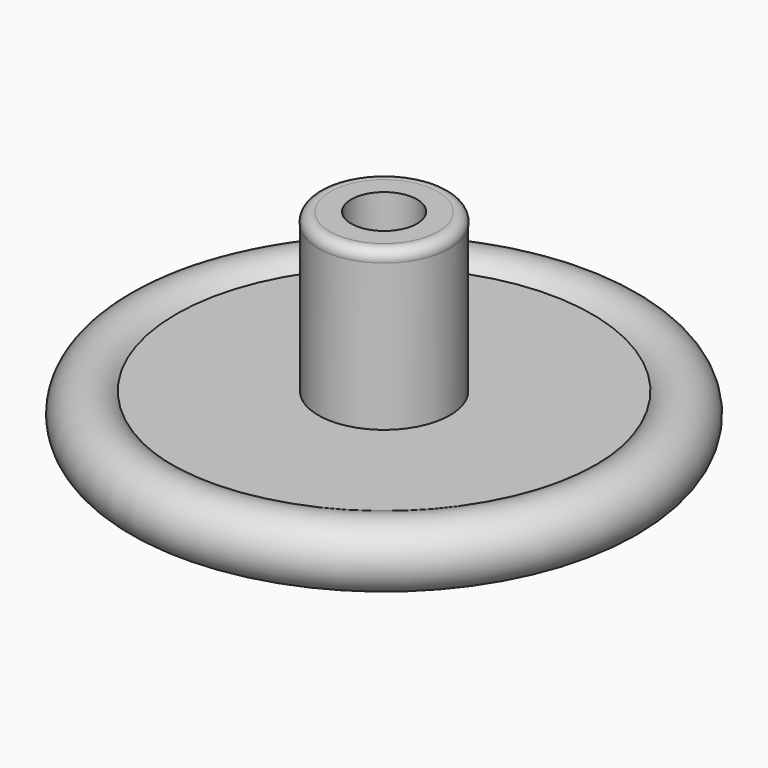
from build123d import *

# Parameters (mm, degrees)
F2_R     = 3.96875
F3_DEPTH = 9.525
F4_R     = 1.5875
F5_DEPTH = 20.6375


# Not quite as in the source:
# - a length typed as a fraction of an inch, garbled in the dataset ("3 / 203.2 mm" for 3/8 in), is restored


with BuildPart() as f1:
    # F0 (on Front) → F1 (revolve)
    with BuildSketch(Plane.XZ):
        with BuildLine():
            Line((0, 30.1625), (0, 0))
            Line((0, 0), (5.2339527756, 0))
            ThreePointArc((5.2339527756, 0), (6.9300739719, 1.2963017107), (7.94385, 3.17499365))
            Line((7.94385, 3.17499365), (7.9375, 6.3499873))
            Line((7.9375, 6.3499873), (25.0110084837, 6.3499873))
            ThreePointArc((25.0110084837, 6.3499873), (31.8322699863, 8.6224170081), (25.0874177301, 11.1125))
            Line((25.0874177301, 11.1125), (7.9375, 11.1125))
            Line((7.9375, 11.1125), (7.9375, 28.8007091731))
            ThreePointArc((7.9375, 28.8007091731), (7.6114687199, 29.8820156927), (6.517462898, 30.1625))
            Line((6.517462898, 30.1625), (0, 30.1625))
        make_face()
    revolve(axis=Axis((0, 0, 15.08125), (0, 0, 1)))

    # F2 (on face) → F3 (cut)
    with BuildSketch(Plane.XY.offset(30.1625)):
        Circle(F2_R)
    extrude(amount=-F3_DEPTH, mode=Mode.SUBTRACT)

    # F4 (on face) → F5 (cut)
    with BuildSketch(Plane(origin=(0, 0, 0), x_dir=(1, 0, 0), z_dir=(0, 0, -1))):
        Circle(F4_R)
    extrude(amount=-F5_DEPTH, mode=Mode.SUBTRACT)


solid = f1.part
